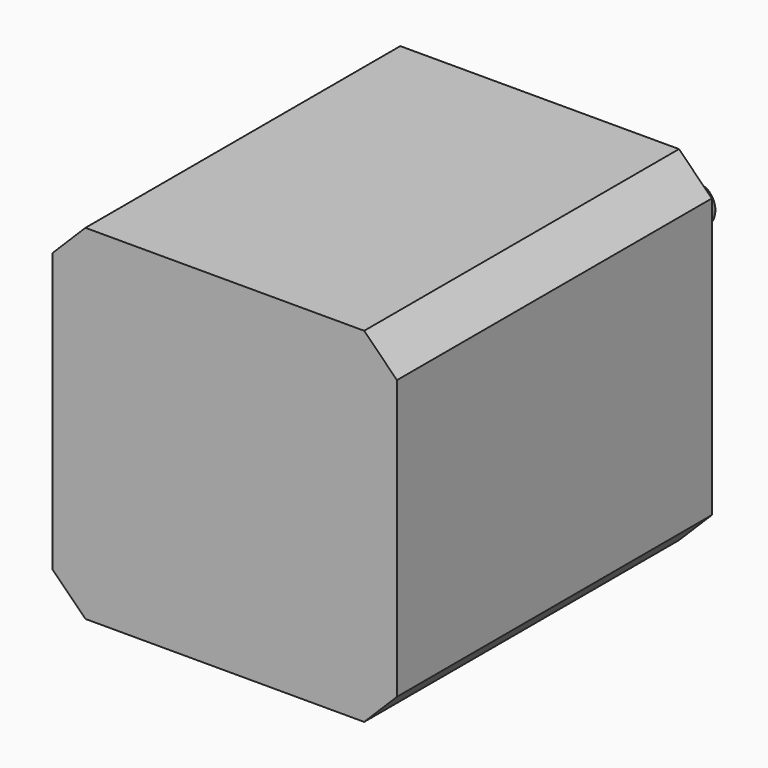
from build123d import *

# Parameters (mm, degrees)
F0_R        = 1.5
F1_DEPTH    = 48
F2_DEPTH    = 4.5
F3_R        = 11
F4_DEPTH    = 2
F5_R        = 2.5
F6_DEPTH    = 22
F8_DEPTH    = 15
F9_T2_ANGLE = 261.8553336274
F9_T4_ANGLE = 81.7820018858


# Not quite as in the source:
# - a fillet or chamfer that OpenCascade refuses, or shapes differently, is made with other operations: its cross-section is extruded or revolved along the edge and cut away or added


with BuildPart() as f1:
    # F0 (on Front) → F1 (new body)
    with BuildSketch(Plane.XZ):
        Polygon((-17, -21), (17, -21), (21, -17), (21, 17), (17, 21), (-17, 21), (-21, 17), (-21, -17), align=None)
        with Locations((-15.5, -15.5)):
            Circle(F0_R, mode=Mode.SUBTRACT)
        with Locations((15.5, -15.5)):
            Circle(F0_R, mode=Mode.SUBTRACT)
        with Locations((-15.5, 15.5)):
            Circle(F0_R, mode=Mode.SUBTRACT)
        with Locations((15.5, 15.5)):
            Circle(F0_R, mode=Mode.SUBTRACT)
        with Locations((-15.5, 15.5)):
            Circle(F0_R)
        with Locations((15.5, 15.5)):
            Circle(F0_R)
        with Locations((-15.5, -15.5)):
            Circle(F0_R)
        with Locations((15.5, -15.5)):
            Circle(F0_R)
    extrude(amount=F1_DEPTH)

    # F0 (on Front) → F2 (cut)
    with BuildSketch(Plane.XZ):
        with Locations((-15.5, 15.5)):
            Circle(F0_R)
        with Locations((-15.5, -15.5)):
            Circle(F0_R)
        with Locations((15.5, 15.5)):
            Circle(F0_R)
        with Locations((15.5, -15.5)):
            Circle(F0_R)
    extrude(amount=F2_DEPTH, mode=Mode.SUBTRACT)

    # F3 (on face) → F4 (join)
    with BuildSketch(Plane.XZ):
        Circle(F3_R)
    extrude(amount=-F4_DEPTH)


with BuildPart() as f6:
    # F5 (on face) → F6 (new body)
    with BuildSketch(Plane(origin=(0, 2, 0), x_dir=(-1, 0, 0), z_dir=(0, 1, 0))):
        Circle(F5_R)
    extrude(amount=F6_DEPTH)

    # F7 (on face) → F8 (cut)
    with BuildSketch(Plane(origin=(0, 24, 0), x_dir=(-1, 0, 0), z_dir=(0, 1, 0))):
        with BuildLine():
            ThreePointArc((1.5, 2), (0, 2.5), (-1.5, 2))
            Line((-1.5, 2), (1.5, 2))
        make_face()
    extrude(amount=-F8_DEPTH, mode=Mode.SUBTRACT)

    # F9: fillet of radius 0.5 on 2 edges, made by hand

    # F9_s1 → F9_t2 (revolve, cut)
    with BuildSketch(Plane(origin=(0, 0, 0), x_dir=(0, 1, 0), z_dir=(-0.9899135138, 0, 0.141672987))):
        with BuildLine():
            ThreePointArc((23.5, -2.5), (23.8535533906, -2.3535533906), (24, -2))
            Line((24, -2), (24, -2.5))
            Line((24, -2.5), (23.5, -2.5))
        make_face()
    revolve(axis=Axis((0, 24, 0), (0, 1, 0)), revolution_arc=F9_T2_ANGLE, mode=Mode.SUBTRACT)

    # F9_s3 → F9_t4 (revolve, cut)
    with BuildSketch(Plane.XY):
        with BuildLine():
            ThreePointArc((-2.5, 23.5), (-2.3535533906, 23.8535533906), (-2, 24))
            Line((-2, 24), (-2.5, 24))
            Line((-2.5, 24), (-2.5, 23.5))
        make_face()
    revolve(axis=Axis((0, 24, 0), (0, 1, 0)), revolution_arc=F9_T4_ANGLE, mode=Mode.SUBTRACT)


solid = Compound([f1.part, f6.part])
